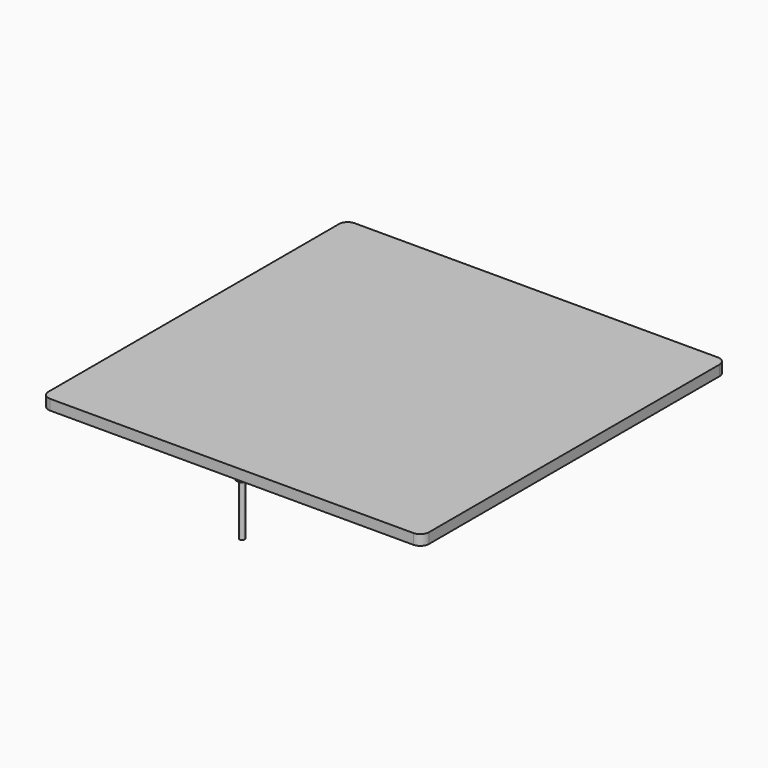
from build123d import *

# Parameters (mm, degrees)
F1_DEPTH = 6
F2_R     = 1.5
F3_DEPTH = 34
F5_DEPTH = 3.9
F6_R     = 2.75
F7_DEPTH = 1.5


with BuildPart() as f1:
    # F0 (on Top) → F1 (new body)
    with BuildSketch(Plane.XY):
        with BuildLine():
            Line((-105, -110), (105, -110))
            ThreePointArc((105, -110), (108.5355339059, -108.5355339059), (110, -105))
            Line((110, -105), (110, 105))
            ThreePointArc((110, 105), (108.5355339059, 108.5355339059), (105, 110))
            Line((105, 110), (-105, 110))
            ThreePointArc((-105, 110), (-108.5355339059, 108.5355339059), (-110, 105))
            Line((-110, 105), (-110, -105))
            ThreePointArc((-110, -105), (-108.5355339059, -108.5355339059), (-105, -110))
        make_face()
    extrude(amount=F1_DEPTH)

    # F2 (on Top) → F3 (join)
    with BuildSketch(Plane.XY):
        with Locations((0, -102.5)):
            Circle(F2_R)
        with Locations((-60, 102)):
            Circle(F2_R)
        with Locations((60, 102)):
            Circle(F2_R)
    extrude(amount=-F3_DEPTH)

    # F4 (on Top) → F5 (join)
    with BuildSketch(Plane.XY):
        Polygon((-1.625, -105.3145825623), (1.625, -105.3145825623), (3.25, -102.5), (1.625, -99.6854174377), (-1.625, -99.6854174377), (-3.25, -102.5), align=None)
        Polygon((58.375, 104.8145825623), (56.75, 102), (58.375, 99.1854174377), (61.625, 99.1854174377), (63.25, 102), (61.625, 104.8145825623), align=None)
        Polygon((-58.375, 104.8145825623), (-61.625, 104.8145825623), (-63.25, 102), (-61.625, 99.1854174377), (-58.375, 99.1854174377), (-56.75, 102), align=None)
    extrude(amount=-F5_DEPTH)


with BuildPart() as f7:
    # F6 (on face) → F7 (new body)
    with BuildSketch(Plane(origin=(0, 0, 0), x_dir=(1, 0, 0), z_dir=(0, 0, -1))):
        Polygon((-35, 100), (-100, 100), (-100, -100), (-79, -100), (-74, -95), (-34, -95), (-29, -100), (-25, -100), (-25, -110), (0, -110), (0, 95), (-30, 95), align=None)
        with Locations((-94.5, -94.5)):
            Circle(F6_R, mode=Mode.SUBTRACT)
        with Locations((-94.5, 94.5)):
            Circle(F6_R, mode=Mode.SUBTRACT)
    extrude(amount=F7_DEPTH)

    # F8: F7 across plane


with BuildPart() as f7_1:
    add(f7.part)
    add(f7.part.mirror(Plane.YZ))


solid = Compound([f1.part, f7_1.part])
